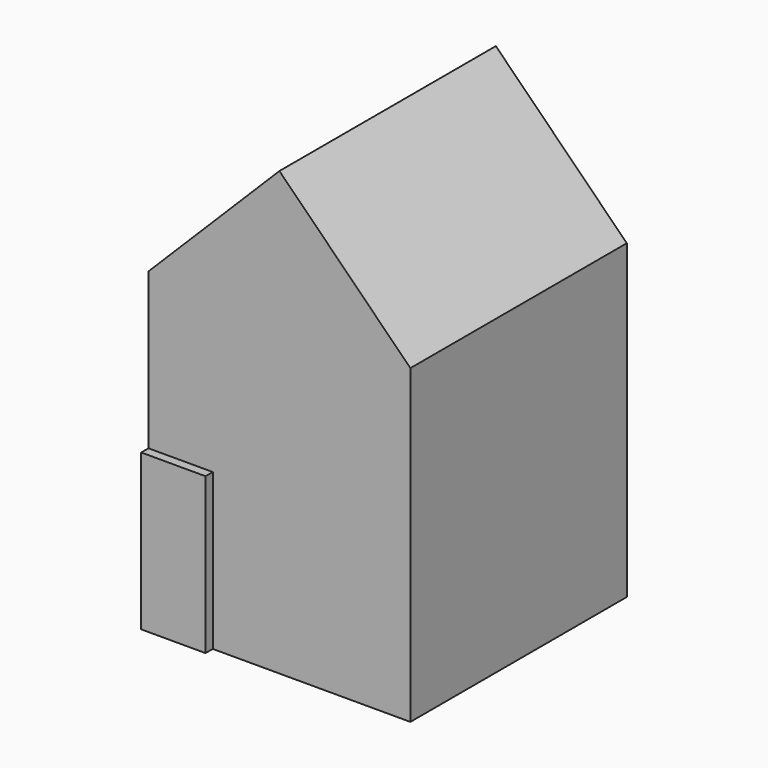
from build123d import *

# Parameters (mm, degrees)
F0_W        = 88.978625834
F0_H        = 91.9070094824
F1_DEPTH    = 92.0228585601
F2_W        = 88.978625834
F2_H        = 91.9070094824
F3_DEPTH    = 64.5945444703
F4_T1_DEPTH = 353.1900010597
F5_W        = 26.5779765323
F5_H        = 57.0915937424
F6_DEPTH    = 3.2936800271
F8_W        = 21.8550208956
F8_H        = 52.9087015152
F9_DEPTH    = 3.0834991485
F10_R       = 12.2707310255
F11_DEPTH   = 1.7256960273
F12_DEPTH   = 0.6503686309


# Not quite as in the source:
# - a fillet or chamfer that OpenCascade refuses, or shapes differently, is made with other operations: its cross-section is extruded or revolved along the edge and cut away or added


with BuildPart() as f1:
    # F0 (on Top) → F1 (new body)
    with BuildSketch(Plane.XY):
        with Locations((-1.1190511286, 2.2303946316)):
            Rectangle(F0_W, F0_H)
    extrude(amount=F1_DEPTH)

    # F2 (on face) → F3 (join)
    with BuildSketch(Plane.XY.offset(92.0228585601)):
        with Locations((-1.1190511286, 2.2303946316)):
            Rectangle(F2_W, F2_H)
    extrude(amount=F3_DEPTH)

    # F4: chamfer of 50.8 on 2 edges, made by hand

    # F4_s2 → F4_t1 (cut)
    with BuildSketch(Plane.XZ.offset(-178.8253951615)):
        Polygon((-45.6083640456, 105.8174030304), (5.1916359544, 156.6174030304), (-45.6083640456, 156.6174030304), align=None)
        Polygon((43.3702617884, 105.8174030304), (-7.4297382116, 156.6174030304), (43.3702617884, 156.6174030304), align=None)
    extrude(amount=F4_T1_DEPTH, mode=Mode.SUBTRACT)

    # F5 (on face) → F6 (join)
    with BuildSketch(Plane(origin=(0, 48.1838993728, 0), x_dir=(-1, 0, 0), z_dir=(0, 1, 0))):
        with Locations((6.6281720065, 28.5457968712)):
            Rectangle(F5_W, F5_H)
    extrude(amount=F6_DEPTH)

    # F8 (on face) → F9 (join)
    with BuildSketch(Plane.XZ.offset(43.7231101096)):
        with Locations((-34.6808535978, 26.4543507576)):
            Rectangle(F8_W, F8_H)
    extrude(amount=F9_DEPTH)

    # F10 (on face) → F11 (join)
    with BuildSketch(Plane(origin=(0, 48.1838993728, 0), x_dir=(-1, 0, 0), z_dir=(0, 1, 0))):
        with Locations((0, 125.5997568369)):
            Circle(F10_R)
    extrude(amount=F11_DEPTH)

    # F12 (add): a face of the model
    f12_faces = [f1.faces().sort_by_distance(p)[0] for p in [
        (0, 49.9095954001, 125.5997568369),
    ]]
    extrude(f12_faces, amount=F12_DEPTH)


solid = f1.part
